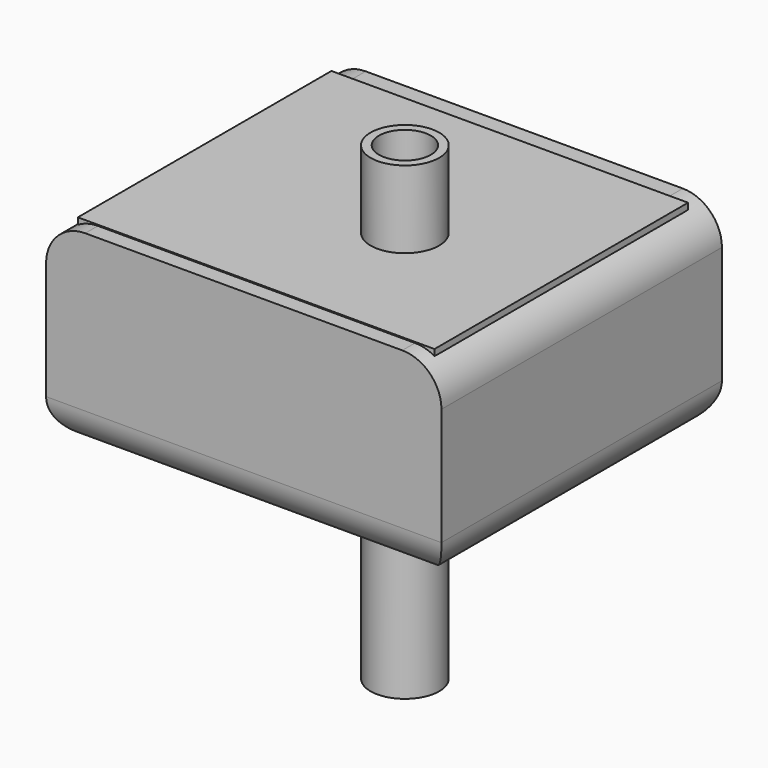
from build123d import *

# Parameters (mm, degrees)
F0_W           = 51.3226017356
F0_H           = 45.5124992877
F1_DEPTH       = 25.4
F2_T           = -2.54
F3_R           = 5.08
F4_W           = 46.2916959077
F4_H           = 2.1475534886
F5_DEPTH       = 23.114
F5_DEPTH_BACK  = 18.034
F6_R           = 6.2989363063
F7_DEPTH       = 25.4
F7_DEPTH_BACK  = 36.83
F8_R           = 4.4507292133
F9_DEPTH       = 35.56
F9_DEPTH_BACK  = 25.4
F10_R          = 3.3711078554
F11_DEPTH      = 27.686
F11_DEPTH_BACK = 52.2224
F12_T4_DEPTH   = 70.9124992877
F12_T10_DEPTH  = 70.9124992877
F12_T16_DEPTH  = 70.9124992877
F12_T23_DEPTH  = 70.9124992877
F12_T29_DEPTH  = 70.9124992877
F12_T35_DEPTH  = 70.9124992877
F12_T41_DEPTH  = 70.9124992877
F12_T47_DEPTH  = 70.9124992877
F12_T54_DEPTH  = 70.9124992877
F12_T60_DEPTH  = 70.9124992877


# Not quite as in the source:
# - a fillet or chamfer that OpenCascade refuses, or shapes differently, is made with other operations: its cross-section is extruded or revolved along the edge and cut away or added


with BuildPart() as f1:
    # F0 (on Top) → F1 (new body)
    with BuildSketch(Plane.XY):
        with Locations((-0.7262639701, -2.4208771065)):
            Rectangle(F0_W, F0_H)
    extrude(amount=F1_DEPTH)

    # F2
    f2_openings = [f1.faces().sort_by_distance(p)[0] for p in [
        (-0.726264, -2.420877, 25.4),
    ]]
    offset(amount=F2_T, openings=f2_openings)

    # F3
    f3_edges = [f1.edges().sort_by_distance(p)[0] for p in [
        (-0.726264, -25.177127, 0),
        (-26.387565, -2.420877, 0),
        (-0.726264, 17.795373, 2.54),
        (22.395037, -2.420877, 2.54),
        (-0.726264, 20.335373, 0),
        (24.935037, -2.420877, 0),
    ]]
    fillet(f3_edges, radius=F3_R)

    # F4 (on Front) → F5 (join, two sides)
    with BuildSketch(Plane.XZ) as f5_sk:
        with Locations((-0.7661757991, 24.4599720463)):
            Rectangle(F4_W, F4_H)
    extrude(amount=F5_DEPTH)
    extrude(f5_sk.sketch, amount=-F5_DEPTH_BACK)

    # F6 (on Top) → F7 (cut, two sides)
    with BuildSketch(Plane.XY) as f7_sk:
        with Locations((-8.230984211, 5.3259306587)):
            Circle(F6_R)
    extrude(amount=F7_DEPTH, mode=Mode.SUBTRACT)
    extrude(f7_sk.sketch, amount=-F7_DEPTH_BACK, mode=Mode.SUBTRACT)

    # F8 (on Top) → F9 (join, two sides)
    with BuildSketch(Plane.XY) as f9_sk:
        with Locations((4.1154921055, -5.0838431343)):
            Circle(F8_R)
    extrude(amount=F9_DEPTH)
    extrude(f9_sk.sketch, amount=-F9_DEPTH_BACK)

    # F10 (on Top) → F11 (cut, two sides)
    with BuildSketch(Plane.XY) as f11_sk:
        with Locations((4.1154921055, -5.0838431343)):
            Circle(F10_R)
    extrude(amount=-F11_DEPTH, mode=Mode.SUBTRACT)
    extrude(f11_sk.sketch, amount=F11_DEPTH_BACK, mode=Mode.SUBTRACT)

    # F12: fillet of radius 5.08 on 2 edges, made by hand


with BuildPart() as f12_tool2:
    # F12_s3 → F12_t4 (new body)
    with BuildSketch(Plane.XZ.offset(37.8771267503)):
        with BuildLine():
            ThreePointArc((24.9350368977, 20.32), (23.4471393461, 23.9121024484), (19.8550368977, 25.4))
            Line((19.8550368977, 25.4), (24.9350368977, 25.4))
            Line((24.9350368977, 25.4), (24.9350368977, 20.32))
        make_face()
    extrude(amount=-F12_T4_DEPTH)

    split(bisect_by=Plane.YZ.offset(22.3796721548), keep=Keep.TOP)

    split(bisect_by=Plane.XZ.offset(23.114), keep=Keep.TOP)


with BuildPart() as f1_1:
    add(f1.part)

    # F12_t1: cut F12_tool2
    add(f12_tool2.part, mode=Mode.SUBTRACT)


with BuildPart() as f12_tool8:
    # F12_s9 → F12_t10 (new body)
    with BuildSketch(Plane.XZ.offset(37.8771267503)):
        with BuildLine():
            ThreePointArc((24.9350368977, 20.32), (23.4471393461, 23.9121024484), (19.8550368977, 25.4))
            Line((19.8550368977, 25.4), (24.9350368977, 25.4))
            Line((24.9350368977, 25.4), (24.9350368977, 20.32))
        make_face()
    extrude(amount=-F12_T10_DEPTH)

    split(bisect_by=Plane.YZ.offset(22.3796721548), keep=Keep.BOTTOM)

    split(bisect_by=Plane.XZ.offset(23.114), keep=Keep.TOP)


with BuildPart() as f1_2:
    add(f1_1.part)

    # F12_t7: cut F12_tool8
    add(f12_tool8.part, mode=Mode.SUBTRACT)


with BuildPart() as f12_tool14:
    # F12_s15 → F12_t16 (new body)
    with BuildSketch(Plane.XZ.offset(37.8771267503)):
        with BuildLine():
            ThreePointArc((24.9350368977, 20.32), (23.4471393461, 23.9121024484), (19.8550368977, 25.4))
            Line((19.8550368977, 25.4), (24.9350368977, 25.4))
            Line((24.9350368977, 25.4), (24.9350368977, 20.32))
        make_face()
    extrude(amount=-F12_T16_DEPTH)

    split(bisect_by=Plane.YZ.offset(22.3796721548), keep=Keep.TOP)

    split(bisect_by=Plane.XZ.offset(-18.034), keep=Keep.TOP)

    split(bisect_by=Plane.XZ.offset(23.114), keep=Keep.BOTTOM)


with BuildPart() as f1_3:
    add(f1_2.part)

    # F12_t13: cut F12_tool14
    add(f12_tool14.part, mode=Mode.SUBTRACT)


with BuildPart() as f12_tool21:
    # F12_s22 → F12_t23 (new body)
    with BuildSketch(Plane.XZ.offset(37.8771267503)):
        with BuildLine():
            ThreePointArc((24.9350368977, 20.32), (23.4471393461, 23.9121024484), (19.8550368977, 25.4))
            Line((19.8550368977, 25.4), (24.9350368977, 25.4))
            Line((24.9350368977, 25.4), (24.9350368977, 20.32))
        make_face()
    extrude(amount=-F12_T23_DEPTH)

    split(bisect_by=Plane.YZ.offset(22.3796721548), keep=Keep.TOP)

    split(bisect_by=Plane.XZ.offset(-18.034), keep=Keep.BOTTOM)


with BuildPart() as f1_4:
    add(f1_3.part)

    # F12_t20: cut F12_tool21
    add(f12_tool21.part, mode=Mode.SUBTRACT)


with BuildPart() as f12_tool27:
    # F12_s28 → F12_t29 (new body)
    with BuildSketch(Plane.XZ.offset(37.8771267503)):
        with BuildLine():
            ThreePointArc((24.9350368977, 20.32), (23.4471393461, 23.9121024484), (19.8550368977, 25.4))
            Line((19.8550368977, 25.4), (24.9350368977, 25.4))
            Line((24.9350368977, 25.4), (24.9350368977, 20.32))
        make_face()
    extrude(amount=-F12_T29_DEPTH)

    split(bisect_by=Plane.YZ.offset(22.3796721548), keep=Keep.BOTTOM)

    split(bisect_by=Plane.XZ.offset(-18.034), keep=Keep.BOTTOM)


with BuildPart() as f1_5:
    add(f1_4.part)

    # F12_t26: cut F12_tool27
    add(f12_tool27.part, mode=Mode.SUBTRACT)


with BuildPart() as f12_tool33:
    # F12_s34 → F12_t35 (new body)
    with BuildSketch(Plane.XZ.offset(-33.0353725374)):
        with BuildLine():
            ThreePointArc((-21.3075648379, 25.4), (-24.8996672864, 23.9121024484), (-26.3875648379, 20.32))
            Line((-26.3875648379, 20.32), (-26.3875648379, 25.4))
            Line((-26.3875648379, 25.4), (-21.3075648379, 25.4))
        make_face()
    extrude(amount=F12_T35_DEPTH)

    split(bisect_by=Plane.XZ.offset(-18.034), keep=Keep.BOTTOM)

    split(bisect_by=Plane.YZ.offset(-23.9120237529), keep=Keep.TOP)


with BuildPart() as f1_6:
    add(f1_5.part)

    # F12_t32: cut F12_tool33
    add(f12_tool33.part, mode=Mode.SUBTRACT)


with BuildPart() as f12_tool39:
    # F12_s40 → F12_t41 (new body)
    with BuildSketch(Plane.XZ.offset(-33.0353725374)):
        with BuildLine():
            ThreePointArc((-21.3075648379, 25.4), (-24.8996672864, 23.9121024484), (-26.3875648379, 20.32))
            Line((-26.3875648379, 20.32), (-26.3875648379, 25.4))
            Line((-26.3875648379, 25.4), (-21.3075648379, 25.4))
        make_face()
    extrude(amount=F12_T41_DEPTH)

    split(bisect_by=Plane.XZ.offset(-18.034), keep=Keep.BOTTOM)

    split(bisect_by=Plane.YZ.offset(-23.9120237529), keep=Keep.BOTTOM)


with BuildPart() as f1_7:
    add(f1_6.part)

    # F12_t38: cut F12_tool39
    add(f12_tool39.part, mode=Mode.SUBTRACT)


with BuildPart() as f12_tool45:
    # F12_s46 → F12_t47 (new body)
    with BuildSketch(Plane.XZ.offset(-33.0353725374)):
        with BuildLine():
            ThreePointArc((-21.3075648379, 25.4), (-24.8996672864, 23.9121024484), (-26.3875648379, 20.32))
            Line((-26.3875648379, 20.32), (-26.3875648379, 25.4))
            Line((-26.3875648379, 25.4), (-21.3075648379, 25.4))
        make_face()
    extrude(amount=F12_T47_DEPTH)

    split(bisect_by=Plane.XZ.offset(-18.034), keep=Keep.TOP)

    split(bisect_by=Plane.YZ.offset(-23.9120237529), keep=Keep.BOTTOM)

    split(bisect_by=Plane.XZ.offset(23.114), keep=Keep.BOTTOM)


with BuildPart() as f1_8:
    add(f1_7.part)

    # F12_t44: cut F12_tool45
    add(f12_tool45.part, mode=Mode.SUBTRACT)


with BuildPart() as f12_tool52:
    # F12_s53 → F12_t54 (new body)
    with BuildSketch(Plane.XZ.offset(-33.0353725374)):
        with BuildLine():
            ThreePointArc((-21.3075648379, 25.4), (-24.8996672864, 23.9121024484), (-26.3875648379, 20.32))
            Line((-26.3875648379, 20.32), (-26.3875648379, 25.4))
            Line((-26.3875648379, 25.4), (-21.3075648379, 25.4))
        make_face()
    extrude(amount=F12_T54_DEPTH)

    split(bisect_by=Plane.YZ.offset(-23.9120237529), keep=Keep.TOP)

    split(bisect_by=Plane.XZ.offset(23.114), keep=Keep.TOP)


with BuildPart() as f1_9:
    add(f1_8.part)

    # F12_t51: cut F12_tool52
    add(f12_tool52.part, mode=Mode.SUBTRACT)


with BuildPart() as f12_tool58:
    # F12_s59 → F12_t60 (new body)
    with BuildSketch(Plane.XZ.offset(-33.0353725374)):
        with BuildLine():
            ThreePointArc((-21.3075648379, 25.4), (-24.8996672864, 23.9121024484), (-26.3875648379, 20.32))
            Line((-26.3875648379, 20.32), (-26.3875648379, 25.4))
            Line((-26.3875648379, 25.4), (-21.3075648379, 25.4))
        make_face()
    extrude(amount=F12_T60_DEPTH)

    split(bisect_by=Plane.YZ.offset(-23.9120237529), keep=Keep.BOTTOM)

    split(bisect_by=Plane.XZ.offset(23.114), keep=Keep.TOP)


with BuildPart() as f1_10:
    add(f1_9.part)

    # F12_t57: cut F12_tool58
    add(f12_tool58.part, mode=Mode.SUBTRACT)


solid = f1_10.part
